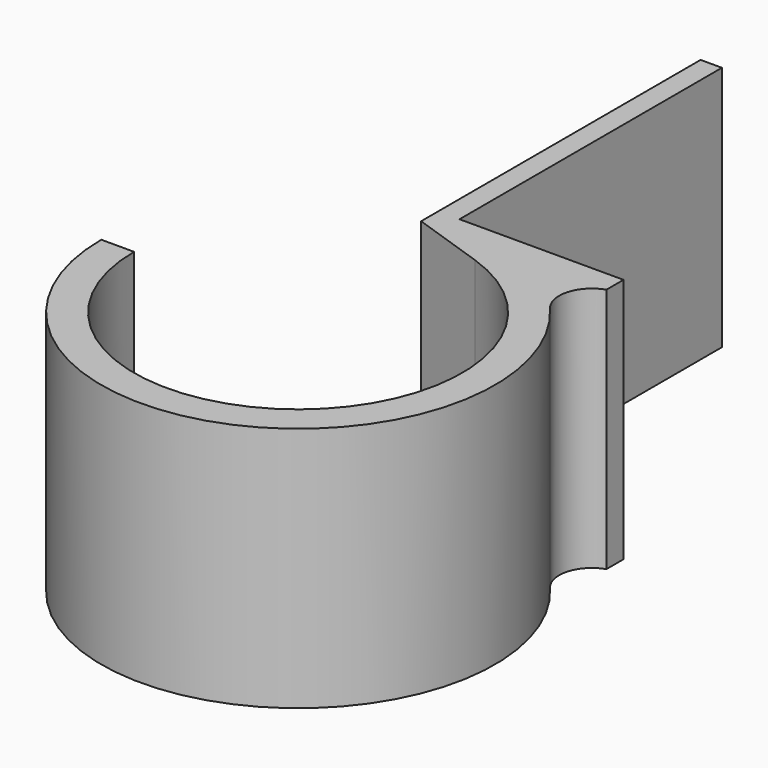
from build123d import *

# Parameters (mm, degrees)
F1_DEPTH    = 19.05
F2_T1_DEPTH = 19.05


# Not quite as in the source:
# - a fillet or chamfer that OpenCascade refuses, or shapes differently, is made with other operations: its cross-section is extruded or revolved along the edge and cut away or added


with BuildPart() as f1:
    # F0 (on Top) → F1 (new body)
    with BuildSketch(Plane.XY):
        Polygon((12.7, 0), (0, 0), (0, -1.651), (6.35, -1.651), (12.7, -1.651), align=None)
        Polygon((0, -1.651), (0, 0), (0, 25.4), (-1.651, 25.4), (-1.651, -1.651), align=None)
        with BuildLine():
            Line((6.35, -1.651), (0, -1.651))
            Line((0, -1.651), (-1.651, -1.651))
            Line((-1.651, -1.651), (4.0781423077, -3.5935831818))
            ThreePointArc((4.0781423077, -3.5935831818), (7.3992429576, -25.9428798508), (-12.7, -15.621))
            Line((-12.7, -15.621), (-15.24, -15.621))
            ThreePointArc((-15.24, -15.621), (7.485390628, -28.8960339791), (7.8868408329, -2.5804731058))
            Line((7.8868408329, -2.5804731058), (6.35, -1.651))
        make_face()
    extrude(amount=F1_DEPTH)

    # F2: fillet of radius 2.54 on 1 edges, made by hand

    # F2_s2 → F2_t1 (join)
    with BuildSketch(Plane.XY):
        with BuildLine():
            ThreePointArc((11.5778863285, -5.7108966623), (11.0593242469, -3.3825527689), (12.7, -1.651))
            Line((12.7, -1.651), (12.619246595, -1.4101787227))
            ThreePointArc((12.619246595, -1.4101787227), (9.525, -1.397), (6.35, -1.397))
            Line((6.35, -1.397), (6.2185526528, -1.8683421149))
            ThreePointArc((6.2185526528, -1.8683421149), (7.7553934856, -2.7978152207), (11.3849215563, -5.8760650512))
            Line((11.3849215563, -5.8760650512), (11.5778863285, -5.7108966623))
        make_face()
    extrude(amount=F2_T1_DEPTH)


solid = f1.part
